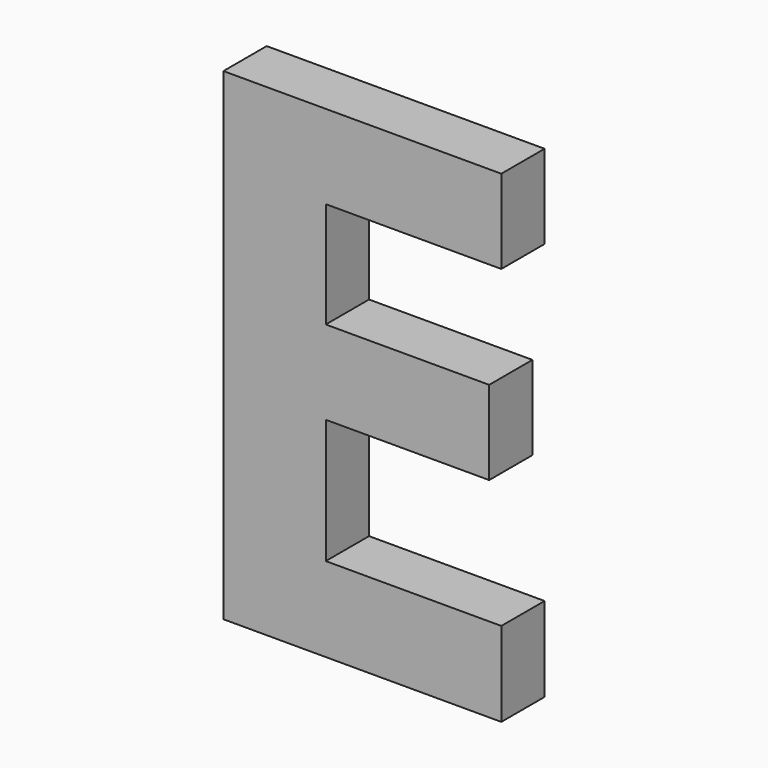
from build123d import *

# Parameters (mm, degrees)
F0_TEXT_SIZE = 62.5
F1_DEPTH     = 5


# Not quite as in the source:
# - Text() gives the source's letters only with a copy of the font that has no kerning and outlines rounded to 1/6400 em; it was checked with that copy


with BuildPart() as f1:
    # F0 (on Front) → F1 (new body)
    with BuildSketch(Plane.XZ):
        with Locations((-68.7890693413, 15.3515624468)):
            Text('E', F0_TEXT_SIZE, font='Open Sans', font_style=FontStyle.BOLD, text_align=(TextAlign.LEFT, TextAlign.BOTTOM))
    extrude(amount=F1_DEPTH)


solid = f1.part
